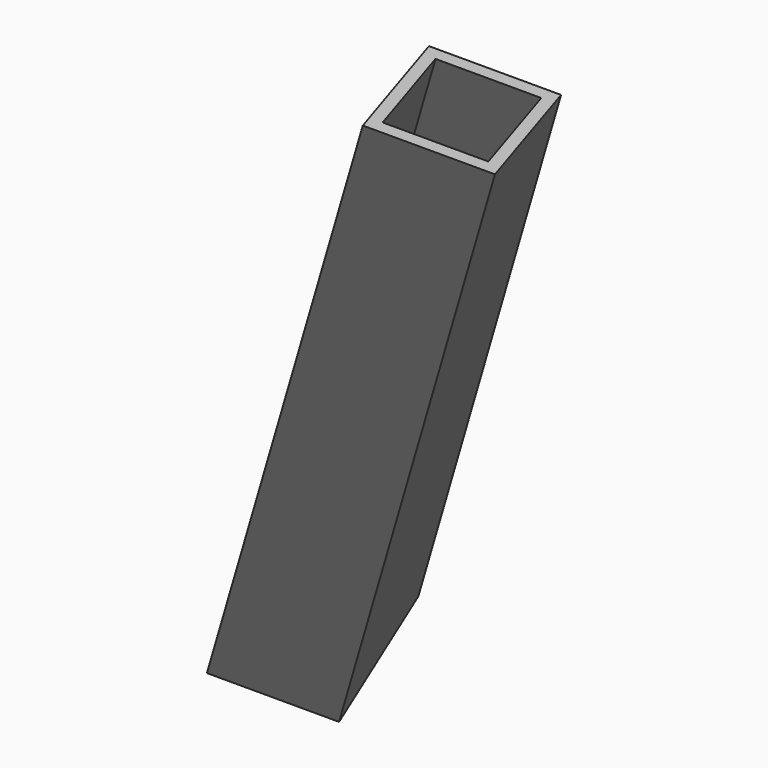
from build123d import *

# Parameters (mm, degrees)
F4_W      = 30
F4_H      = 30
F4_W_2    = 24
F4_H_2    = 24
F5_DEPTH  = 1000
F7_W      = 1359.9022671681
F7_H      = 1462.2605508027
F8_DEPTH  = 477.3996029769
F11_W     = 260.7968747616
F11_H     = 228.6183834076
F12_DEPTH = 46.9924863148
F13_R     = 6.3105959623
F14_DEPTH = 3


with BuildPart() as f5:
    # F4 (on face) → F5 (new body)
    with BuildSketch(Plane(origin=(0, 0, 0), x_dir=(0.8660254038, 0.2753467822, -0.4173537463), z_dir=(0.5, -0.4769146164, 0.7228778933))):
        Rectangle(F4_W, F4_H)
        Rectangle(F4_W_2, F4_H_2, mode=Mode.SUBTRACT)
    extrude(amount=F5_DEPTH)

    # F7 (on offset) → F8 (cut, through all)
    with BuildSketch(Plane.XY.offset(260)):
        with Locations((509.8009683141, -255.676958236)):
            Rectangle(F7_W, F7_H)
    extrude(amount=F8_DEPTH, mode=Mode.SUBTRACT)

    # F11 (on face) → F12 (cut, through all)
    with BuildSketch(Plane(origin=(0, -17.1818181667, 18.1599869076), x_dir=(1, 0, 0), z_dir=(0, -0.6872727267, 0.7263994763))):
        Rectangle(F11_W, F11_H)
    extrude(amount=-F12_DEPTH, mode=Mode.SUBTRACT)

    # F13 (on face) → F14 (cut, through all)
    with BuildSketch(Plane(origin=(0, 12.5206123889, 8.2604034651), x_dir=(-1, 0, 0), z_dir=(0, 0.8347074926, 0.5506935643))):
        with Locations((-16.1834571395, 28.0305700078)):
            Circle(F13_R)
    extrude(amount=-F14_DEPTH, mode=Mode.SUBTRACT)


solid = f5.part
